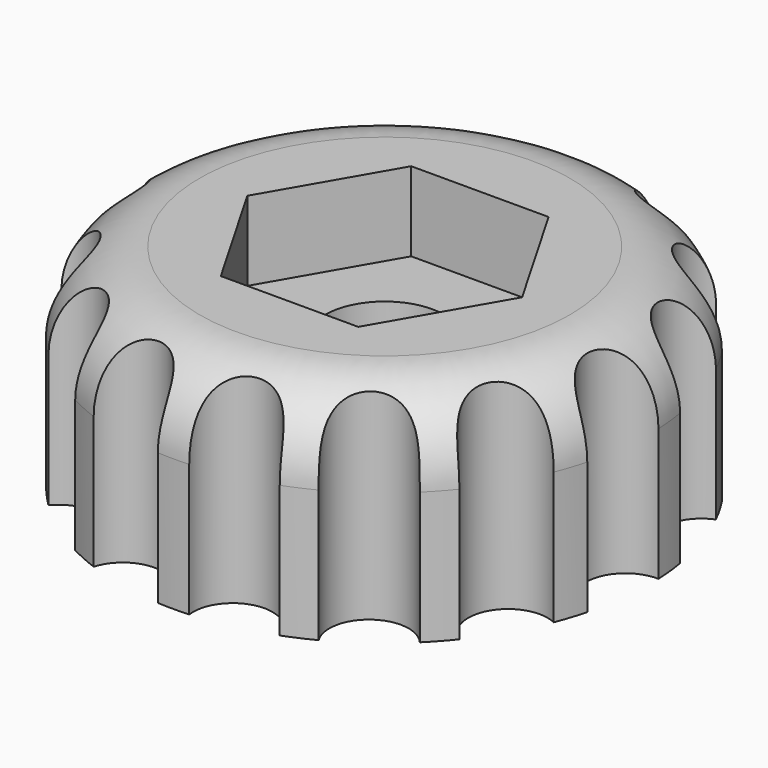
from build123d import *

# Parameters (mm, degrees)
F0_R     = 10
F0_R_2   = 2.25
F1_DEPTH = 8
F4_DEPTH = 3
F5_R     = 3
F7_DEPTH = 25


with BuildPart() as f1:
    # F0 (on Top) → F1 (new body)
    with BuildSketch(Plane.XY):
        Circle(F0_R)
        Circle(F0_R_2, mode=Mode.SUBTRACT)
    extrude(amount=F1_DEPTH)

    # F3 (on face) → F4 (cut)
    with BuildSketch(Plane.XY.offset(8)):
        Polygon((-2.5980762114, -4.5), (2.5980762114, -4.5), (5.1961524227, 0), (2.5980762114, 4.5), (-2.5980762114, 4.5), (-5.1961524227, 0), align=None)
    extrude(amount=-F4_DEPTH, mode=Mode.SUBTRACT)

    # F5
    f5_edges = [f1.edges().sort_by_distance(p)[0] for p in [
        (-10, 0, 8),
    ]]
    fillet(f5_edges, radius=F5_R)

    # F6 (on face) → F7 (cut)
    with BuildSketch(Plane.XY.offset(8)):
        with BuildLine():
            ThreePointArc((-8.010565163, 3.0901699437), (-8.2648082106, 3.9256875173), (-8.9413513172, 4.4779723785))
            ThreePointArc((-8.9413513172, 4.4779723785), (-9.510565163, 3.0901699437), (-9.8657912925, 1.6328386853))
            ThreePointArc((-9.8657912925, 1.6328386853), (-8.583969025, 1.9105854418), (-8.010565163, 3.0901699437))
        make_face()
        with BuildLine():
            ThreePointArc((-5.9314482548, 6.6913060636), (-6.0392002093, 7.2495581392), (-6.346975428, 7.7276065451))
            ThreePointArc((-6.346975428, 7.7276065451), (-7.4314482548, 6.6913060636), (-8.3487134958, 5.5044511956))
            ThreePointArc((-8.3487134958, 5.5044511956), (-6.7703498739, 5.3448481434), (-5.9314482548, 6.6913060636))
        make_face()
        with BuildLine():
            ThreePointArc((-9.3107138302, -3.6483705913), (-8.6602540378, -5), (-7.8149385296, -6.2391294087))
            ThreePointArc((-7.8149385296, -6.2391294087), (-7.3339861044, -5.700723461), (-7.1602540378, -5))
            ThreePointArc((-7.1602540378, -5), (-7.8620340458, -3.730021715), (-9.3107138302, -3.6483705913))
        make_face()
        with BuildLine():
            ThreePointArc((-9.989686334, 0.4540561065), (-9.9452189537, -1.0452846327), (-9.6769841469, -2.5211064676))
            ThreePointArc((-9.6769841469, -2.5211064676), (-8.7936217563, -2.0064422134), (-8.4452189537, -1.0452846327))
            ThreePointArc((-8.4452189537, -1.0452846327), (-8.9003986511, 0.0309823116), (-9.989686334, 0.4540561065))
        make_face()
        with BuildLine():
            ThreePointArc((-7.02183432, -7.1199608694), (-5.8778525229, -8.0901699437), (-4.6016190441, -8.8783501943))
            ThreePointArc((-4.6016190441, -8.8783501943), (-4.4348781264, -8.4998343074), (-4.3778525229, -8.0901699437))
            ThreePointArc((-4.3778525229, -8.0901699437), (-5.3611188854, -6.6819844631), (-7.02183432, -7.1199608694))
        make_face()
        with BuildLine():
            ThreePointArc((-3.5188158645, -9.3604452304), (-2.0791169082, -9.7814760073), (-0.5926378214, -9.9824235741))
            ThreePointArc((-0.5926378214, -9.9824235741), (-0.5825009537, -9.8821769752), (-0.5791169082, -9.7814760073))
            ThreePointArc((-0.5791169082, -9.7814760073), (-1.8664533647, -8.2966277938), (-3.5188158645, -9.3604452304))
        make_face()
        with BuildLine():
            ThreePointArc((0.5926378214, -9.9824235741), (2.0791169082, -9.7814760073), (3.5188158645, -9.3604452304))
            ThreePointArc((3.5188158645, -9.3604452304), (1.767249372, -8.3142546062), (0.5926378214, -9.9824235741))
        make_face()
        with BuildLine():
            ThreePointArc((4.6016190441, -8.8783501943), (5.8778525229, -8.0901699437), (7.02183432, -7.1199608694))
            ThreePointArc((7.02183432, -7.1199608694), (4.9961746445, -6.8766444522), (4.6016190441, -8.8783501943))
        make_face()
        with BuildLine():
            ThreePointArc((7.8149385296, -6.2391294087), (8.6602540378, -5), (9.3107138302, -3.6483705913))
            ThreePointArc((9.3107138302, -3.6483705913), (7.3612159322, -4.25), (7.8149385296, -6.2391294087))
        make_face()
        with BuildLine():
            ThreePointArc((9.6769841469, -2.5211064676), (9.9189173166, -1.270857689), (10, 0))
            ThreePointArc((10, 0), (9.997421251, 0.2270866132), (9.989686334, 0.4540561065))
            ThreePointArc((9.989686334, 0.4540561065), (8.4534361106, -0.8884919378), (9.6769841469, -2.5211064676))
        make_face()
        with BuildLine():
            ThreePointArc((8.9413513172, 4.4779723785), (8.0839803885, 2.6266444522), (9.8657912925, 1.6328386853))
            ThreePointArc((9.8657912925, 1.6328386853), (9.510565163, 3.0901699437), (8.9413513172, 4.4779723785))
        make_face()
        with BuildLine():
            ThreePointArc((6.346975428, 7.7276065451), (6.3167310166, 5.6876101541), (8.3487134958, 5.5044511956))
            ThreePointArc((8.3487134958, 5.5044511956), (7.4314482548, 6.6913060636), (6.346975428, 7.7276065451))
        make_face()
        with BuildLine():
            ThreePointArc((2.6551498269, 9.641067337), (3.4572614661, 7.76513639), (5.38806729, 8.4242940879))
            ThreePointArc((5.38806729, 8.4242940879), (4.0673664308, 9.1354545764), (2.6551498269, 9.641067337))
        make_face()
        with BuildLine():
            ThreePointArc((-1.4957753006, 9.8875), (0, 8.5), (1.4957753006, 9.8875))
            ThreePointArc((1.4957753006, 9.8875), (0, 10), (-1.4957753006, 9.8875))
        make_face()
        with BuildLine():
            ThreePointArc((-2.5673664308, 9.1354545764), (-2.5894752125, 9.3920428596), (-2.6551498269, 9.641067337))
            ThreePointArc((-2.6551498269, 9.641067337), (-4.0673664308, 9.1354545764), (-5.38806729, 8.4242940879))
            ThreePointArc((-5.38806729, 8.4242940879), (-3.7006589784, 7.6809699102), (-2.5673664308, 9.1354545764))
        make_face()
    extrude(amount=-F7_DEPTH, mode=Mode.SUBTRACT)


solid = f1.part
